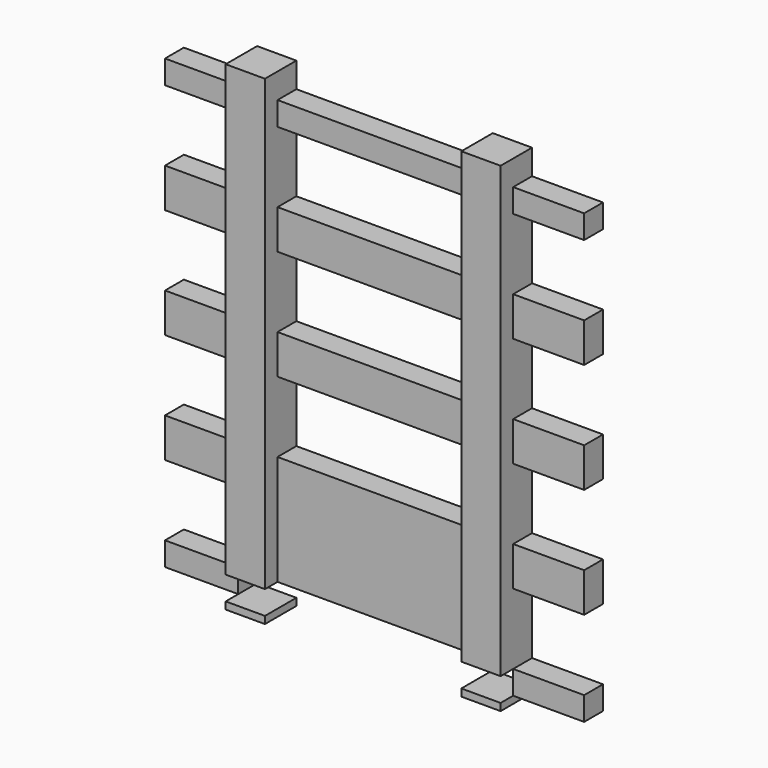
from build123d import *

# Parameters (mm, degrees)
F0_W     = 12.7
F0_H     = 8.135657315
F0_H_2   = 22.86
F0_H_3   = 7.62
F0_H_4   = 12.7
F1_DEPTH = 12.7
F0_H_5   = 2.3344613409
F0_W_2   = 23.6822664738
F2_DEPTH = 7.62
F0_W_3   = 63.5
F0_W_4   = 22.954866147


# Not quite as in the source:
# - a feature names something its author has since deleted; it is built from what else it names


with BuildPart() as f1:
    # F0 (on Front) → F1 (new body)
    with BuildSketch(Plane.XZ):
        with Locations((-41.6535617948, 70.1078286575)):
            Rectangle(F0_W, F0_H)
        with Locations((-41.6535617948, 46.99)):
            Rectangle(F0_W, F0_H_2)
        with Locations((-41.6535617948, 11.43)):
            Rectangle(F0_W, F0_H_2)
        with Locations((-41.6535617948, -24.13)):
            Rectangle(F0_W, F0_H_2)
        with Locations((-41.6535617948, 62.23)):
            Rectangle(F0_W, F0_H_3)
        Polygon((-35.3035617948, -71.12), (-35.3035617948, -67.4191057513), (-35.3035617948, -48.26), (-48.0035617948, -48.26), (-48.0035617948, -67.4191057513), (-48.0035617948, -71.12), align=None)
        with Locations((-41.6535617948, -41.91)):
            Rectangle(F0_W, F0_H_4)
        with Locations((-41.6535617948, -6.35)):
            Rectangle(F0_W, F0_H_4)
        with Locations((-41.6535617948, 29.21)):
            Rectangle(F0_W, F0_H_4)
    extrude(amount=F1_DEPTH)


with BuildPart() as f1b:
    # F0 (on Front) → F1, piece 2 (new body)
    with BuildSketch(Plane.XZ):
        with Locations((34.5464382052, 70.1078286575)):
            Rectangle(F0_W, F0_H)
        with Locations((34.5464382052, 46.99)):
            Rectangle(F0_W, F0_H_2)
        with Locations((34.5464382052, 11.43)):
            Rectangle(F0_W, F0_H_2)
        with Locations((34.5464382052, -24.13)):
            Rectangle(F0_W, F0_H_2)
        with Locations((34.5464382052, 62.23)):
            Rectangle(F0_W, F0_H_3)
        with Locations((34.5464382052, 29.21)):
            Rectangle(F0_W, F0_H_4)
        with Locations((34.5464382052, -6.35)):
            Rectangle(F0_W, F0_H_4)
        with Locations((34.5464382052, -41.91)):
            Rectangle(F0_W, F0_H_4)
        Polygon((40.8964382052, -48.26), (28.1964382052, -48.26), (28.1964382052, -67.4191057513), (28.1964382052, -71.12), (40.8964382052, -71.12), (40.8964382052, -67.4191057513), align=None)
    extrude(amount=F1_DEPTH)


with BuildPart() as f1c:
    # F0 (on Front) → F1, piece 3 (new body)
    with BuildSketch(Plane.XZ):
        with Locations((34.5464382052, -79.9072306705)):
            Rectangle(F0_W, F0_H_5)
    extrude(amount=F1_DEPTH)


with BuildPart() as f1d:
    # F0 (on Front) → F1, piece 4 (new body)
    with BuildSketch(Plane.XZ):
        with Locations((-41.6535617948, -79.9072306705)):
            Rectangle(F0_W, F0_H_5)
    extrude(amount=F1_DEPTH)


with BuildPart() as f2:
    # F0 (on Front) → F2 (new body)
    with BuildSketch(Plane.XZ):
        with Locations((-59.8446950316, 62.23)):
            Rectangle(F0_W_2, F0_H_3)
    extrude(amount=F2_DEPTH)


with BuildPart() as f2b:
    # F0 (on Front) → F2, piece 2 (new body)
    with BuildSketch(Plane.XZ):
        with Locations((-3.5535617948, 62.23)):
            Rectangle(F0_W_3, F0_H_3)
    extrude(amount=F2_DEPTH)


with BuildPart() as f2c:
    # F0 (on Front) → F2, piece 3 (new body)
    with BuildSketch(Plane.XZ):
        with Locations((-59.8446950316, 29.21)):
            Rectangle(F0_W_2, F0_H_4)
    extrude(amount=F2_DEPTH)


with BuildPart() as f2d:
    # F0 (on Front) → F2, piece 4 (new body)
    with BuildSketch(Plane.XZ):
        with Locations((-3.5535617948, 29.21)):
            Rectangle(F0_W_3, F0_H_4)
    extrude(amount=F2_DEPTH)


with BuildPart() as f2e:
    # F0 (on Front) → F2, piece 5 (new body)
    with BuildSketch(Plane.XZ):
        with Locations((-59.8446950316, -6.35)):
            Rectangle(F0_W_2, F0_H_4)
    extrude(amount=F2_DEPTH)


with BuildPart() as f2f:
    # F0 (on Front) → F2, piece 6 (new body)
    with BuildSketch(Plane.XZ):
        with Locations((-3.5535617948, -6.35)):
            Rectangle(F0_W_3, F0_H_4)
    extrude(amount=F2_DEPTH)


with BuildPart() as f2g:
    # F0 (on Front) → F2, piece 7 (new body)
    with BuildSketch(Plane.XZ):
        with Locations((-59.8446950316, -41.91)):
            Rectangle(F0_W_2, F0_H_4)
    extrude(amount=F2_DEPTH)


with BuildPart() as f2h:
    # F0 (on Front) → F2, piece 8 (new body)
    with BuildSketch(Plane.XZ):
        with Locations((-3.5535617948, -41.91)):
            Rectangle(F0_W_3, F0_H_4)
        Polygon((-35.3035617948, -48.26), (-35.3035617948, -67.4191057513), (-35.3035617948, -71.12), (28.1964382052, -71.12), (28.1964382052, -67.4191057513), (28.1964382052, -48.26), align=None)
    extrude(amount=F2_DEPTH)


with BuildPart() as f2i:
    # F0 (on Front) → F2, piece 9 (new body)
    with BuildSketch(Plane.XZ):
        with Locations((-59.8446950316, -74.93)):
            Rectangle(F0_W_2, F0_H_3)
    extrude(amount=F2_DEPTH)


with BuildPart() as f2j:
    # F0 (on Front) → F2, piece 10 (new body)
    with BuildSketch(Plane.XZ):
        with Locations((52.3738712788, -74.93)):
            Rectangle(F0_W_4, F0_H_3)
    extrude(amount=F2_DEPTH)


with BuildPart() as f2k:
    # F0 (on Front) → F2, piece 11 (new body)
    with BuildSketch(Plane.XZ):
        with Locations((52.3738712788, -41.91)):
            Rectangle(F0_W_4, F0_H_4)
    extrude(amount=F2_DEPTH)


with BuildPart() as f2l:
    # F0 (on Front) → F2, piece 12 (new body)
    with BuildSketch(Plane.XZ):
        with Locations((52.3738712788, -6.35)):
            Rectangle(F0_W_4, F0_H_4)
    extrude(amount=F2_DEPTH)


with BuildPart() as f2m:
    # F0 (on Front) → F2, piece 13 (new body)
    with BuildSketch(Plane.XZ):
        with Locations((52.3738712788, 29.21)):
            Rectangle(F0_W_4, F0_H_4)
    extrude(amount=F2_DEPTH)


with BuildPart() as f2n:
    # F0 (on Front) → F2, piece 14 (new body)
    with BuildSketch(Plane.XZ):
        with Locations((52.3738712788, 62.23)):
            Rectangle(F0_W_4, F0_H_3)
    extrude(amount=F2_DEPTH)


solid = Compound([f1.part, f1b.part, f1c.part, f1d.part, f2.part, f2b.part, f2c.part, f2d.part, f2e.part, f2f.part, f2g.part, f2h.part, f2i.part, f2j.part, f2k.part, f2l.part, f2m.part, f2n.part])
